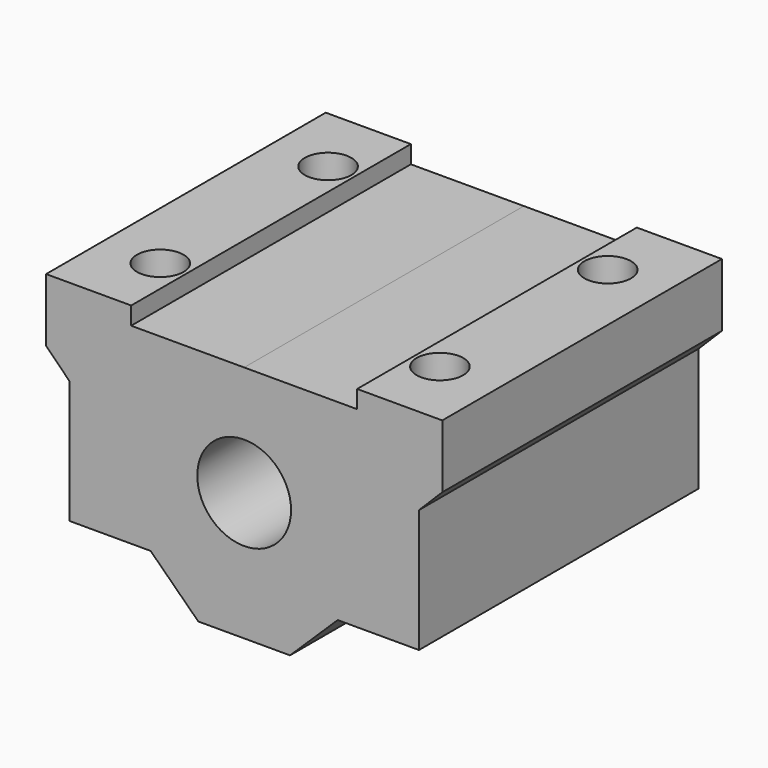
from build123d import *

# Parameters (mm, degrees)
F0_R          = 4.025
F1_DEPTH      = 30
F2_R          = 2
F3_DEPTH      = 10.9999993406
F3_DEPTH_BACK = 25


# Not quite as in the source:
# - ends of sketch curves that miss each other by under 0.0002 mm in the source are joined


with BuildPart() as f1:
    # F0 (on Front) → F1 (new body)
    with BuildSketch(Plane.XZ):
        Polygon((-17, 10.9999990659), (-17, 5.5723366328), (-15, 3.5723366328), (-15, -7.0000008242), (-8.0288857139, -7.0000004412), (-3.9351008678, -11.0000002162), (3.022e-07, -11), (3.9351014722, -10.9999997838), (8.0288857139, -7.0000004412), (15, -7.0000008242), (15, 3.5723366328), (17, 5.5723366328), (17, 10.9999990659), (9.6955373869, 10.9999994673), (9.6955373029, 9.4717088947), (8.4e-08, 9.4717094274), (-9.6955373029, 9.4717088947), (-9.6955373869, 10.9999994673), align=None)
        Circle(F0_R, mode=Mode.SUBTRACT)
    extrude(amount=F1_DEPTH)

    # F2 (on Top) → F3 (cut, two sides)
    with BuildSketch(Plane.XY) as f3_sk:
        with Locations((-12, -6)):
            Circle(F2_R)
        with Locations((-12, -24)):
            Circle(F2_R)
        with Locations((12, -6)):
            Circle(F2_R)
        with Locations((12, -24)):
            Circle(F2_R)
    extrude(amount=F3_DEPTH, mode=Mode.SUBTRACT)
    extrude(f3_sk.sketch, amount=-F3_DEPTH_BACK, mode=Mode.SUBTRACT)


solid = f1.part
